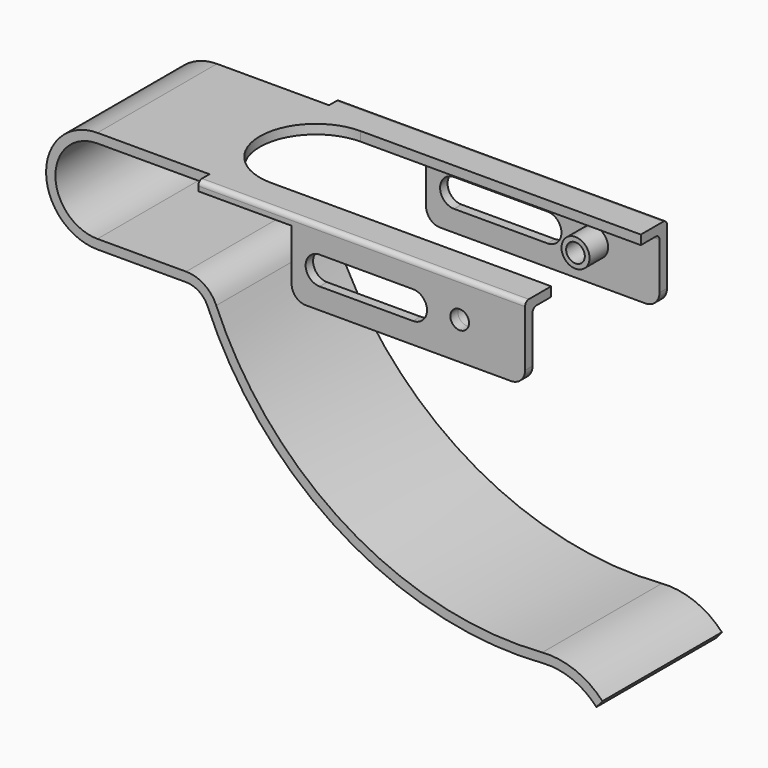
from build123d import *

# Parameters (mm, degrees)
F1_DEPTH  = 16
F2_W      = 70
F2_H      = 3
F3_DEPTH  = 2
F4_W      = 50
F4_H      = 14
F5_DEPTH  = 2
F6_R      = 1
F9_DEPTH  = 4
F11_DEPTH = 38.001
F13_D     = 4
F14_R     = 3
F14_R_2   = 2
F15_DEPTH = 5
F16_R     = 3


# Not quite as in the source:
# - a pattern or mirror of a feature is missing from the dataset's text; its kind, count and spacing are read off the source's solid


with BuildPart() as f1:
    # F0 (on Front) → F1 (new body)
    with BuildSketch(Plane.XZ):
        with BuildLine():
            Line((94, 11), (0, 11))
            ThreePointArc((0, 11), (-11, 0), (0, -11))
            Line((0, -11), (19, -11))
            ThreePointArc((19, -11), (21.7681124643, -11.8361612201), (23.6103896104, -14.064978646))
            ThreePointArc((23.6103896104, -14.064978646), (52.4378053116, -47.6260855158), (95.4479042723, -57.9942665386))
            ThreePointArc((95.4479042723, -57.9942665386), (101.6870615127, -58.9476250352), (106.8734428361, -62.5444881493))
            Line((106.8734428361, -62.5444881493), (108.1694222725, -61))
            ThreePointArc((108.1694222725, -61), (102.3002117906, -57.039668375), (95.2965735981, -56))
            ThreePointArc((95.2965735981, -56), (53.4811996085, -45.9198240056), (25.4545454545, -13.2909701044))
            ThreePointArc((25.4545454545, -13.2909701044), (22.87535745, -10.1706257081), (19, -9))
            Line((19, -9), (0, -9))
            ThreePointArc((0, -9), (-9, 0), (0, 9))
            Line((0, 9), (94, 9))
            Line((94, 9), (94, 11))
        make_face()
    extrude(amount=F1_DEPTH)

    # F2 (on face) → F3 (join)
    with BuildSketch(Plane.XY.offset(11)):
        with Locations((59, -17.5)):
            Rectangle(F2_W, F2_H)
    extrude(amount=-F3_DEPTH)

    # F4 (on face) → F5 (join)
    with BuildSketch(Plane.XZ.offset(19)):
        with Locations((69, 2)):
            Rectangle(F4_W, F4_H)
    extrude(amount=-F5_DEPTH)

    # F6
    f6_edges = [f1.edges().sort_by_distance(p)[0] for p in [
        (59, -19, 11),
        (69, -17, 9),
    ]]
    fillet(f6_edges, radius=F6_R)

    # F7: F1 across plane


with BuildPart() as f1_1:
    add(f1.part)
    add(f1.part.mirror(Plane.XZ))

    # F8 (on face) → F9 (cut)
    with BuildSketch(Plane.XY.offset(11)):
        with BuildLine():
            Line((94, 12), (34, 12))
            ThreePointArc((34, 12), (22, 0), (34, -12))
            Line((34, -12), (94, -12))
            Line((94, -12), (94, 12))
        make_face()
    extrude(amount=-F9_DEPTH, mode=Mode.SUBTRACT)

    # F10 (on face) → F11 (cut, through all)
    with BuildSketch(Plane.XZ.offset(19)):
        with BuildLine():
            ThreePointArc((70, -0.5), (73, 2.5), (70, 5.5))
            Line((70, 5.5), (50, 5.5))
            ThreePointArc((50, 5.5), (47, 2.5), (50, -0.5))
            Line((50, -0.5), (70, -0.5))
        make_face()
    extrude(amount=-F11_DEPTH, mode=Mode.SUBTRACT)

    # F13 (through all)
    with Locations(Plane.XZ.offset(19)):
        with Locations((80, 3)):
            Hole(F13_D / 2)

    # F14 (on face) → F15 (join)
    with BuildSketch(Plane(origin=(0, -17, 0), x_dir=(-1, 0, 0), z_dir=(0, 1, 0))):
        with Locations((-80, 3)):
            Circle(F14_R)
        with Locations((-80, 3)):
            Circle(F14_R_2, mode=Mode.SUBTRACT)
    f15 = extrude(amount=F15_DEPTH)

    # F15_copies: F15 across plane
    add(f15.mirror(Plane.ZX))

    # F16
    f16_edges = [f1_1.edges().sort_by_distance(p)[0] for p in [
        (94, 18, -5),
        (44, 18, -5),
        (94, -18, -5),
        (44, -18, -5),
    ]]
    fillet(f16_edges, radius=F16_R)


solid = f1_1.part
